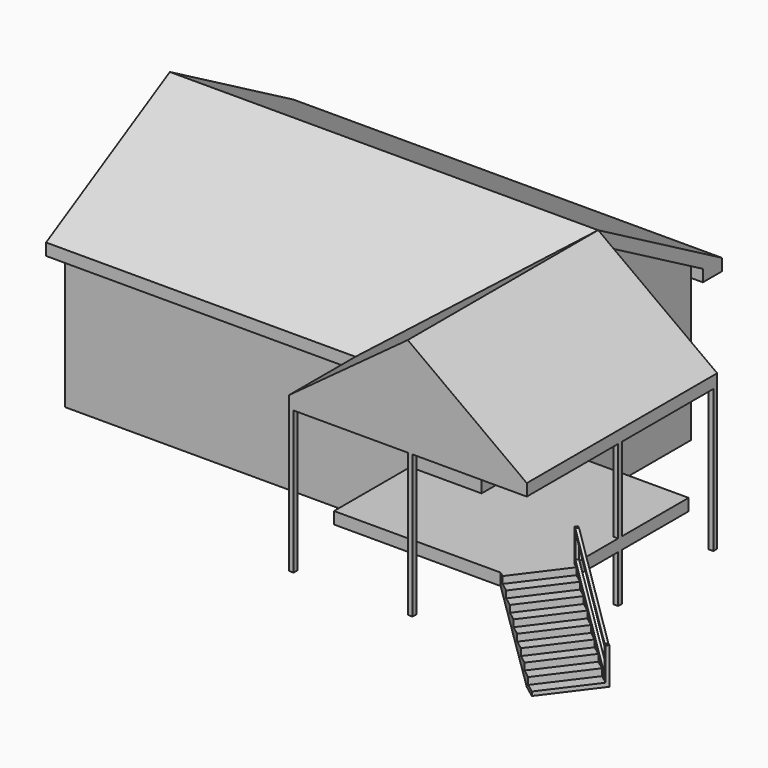
from build123d import *

# Parameters (mm, degrees)
F0_W           = 558.8
F0_H           = 304.8
F1_DEPTH       = 889
F3_DEPTH       = 889
F5_DEPTH       = 25.4
F7_DEPTH       = 330.2
F7_DEPTH_BACK  = 177.8
F8_W           = 10.16
F8_H           = 10.16
F9_DEPTH       = 304.8
F11_DEPTH      = 203.2
F11_DEPTH_BACK = 203.2
F14_DEPTH      = 25.4
F15_W          = 6.35
F15_H          = 127.005368185
F16_DEPTH      = 304.8
F18_DEPTH      = 25.4
F19_DEPTH      = 127
F20_W          = 6.5650812721
F20_H          = 95.2373991132
F21_DEPTH      = 6.35
F22_W          = 6.35
F22_H          = 78.3844
F23_DEPTH      = 6.35
F25_DEPTH      = 6.35
F27_DEPTH      = 6.35


# Not quite as in the source:
# - a feature of the source that left no trace in its solid (it failed there, or was rolled back) is left out


with BuildPart() as f1:
    # F0 (on Right) → F1 (new body)
    with BuildSketch(Plane.YZ):
        with Locations((279.4, -152.4)):
            Rectangle(F0_W, F0_H)
    extrude(amount=F1_DEPTH)

    # F2 (on face) → F3 (join)
    with BuildSketch(Plane(origin=(0, 0, 0), x_dir=(0, -1, 0), z_dir=(-1, 0, 0))):
        Polygon((-609.6, 0), (-558.8, 0), (0, 0), (50.8, 0), (50.8, 25.4), (-279.4, 211.5524560213), (-609.6, 25.4), align=None)
    extrude(amount=-F3_DEPTH)

    # F4 (on face) → F5 (join)
    with BuildSketch(Plane.YZ.offset(889)):
        Polygon((-50.8, 25.4), (-50.8, 0), (0, 0), (0, 25.4), (279.4, 182.9136166334), (558.8, 25.4), (558.8, 0), (609.6, 0), (609.6, 25.4), (279.4, 211.5524560213), align=None)
    extrude(amount=F5_DEPTH)

    # F6 (on face) → F7 (join, two sides)
    with BuildSketch(Plane.XZ.offset(50.8)) as f7_sk:
        Polygon((889, 0), (914.4, 0), (1168.4, 0), (1168.4, 25.4), (914.4, 211.6865664721), (660.4, 25.4), (660.4, 0), align=None)
    extrude(amount=-F7_DEPTH)
    extrude(f7_sk.sketch, amount=F7_DEPTH_BACK)

    # F8 (on face) → F9 (join)
    with BuildSketch(Plane(origin=(0, 0, 0), x_dir=(1, 0, 0), z_dir=(0, 0, -1))):
        with Locations((665.48, 223.52)):
            Rectangle(F8_W, F8_H)
        with Locations((1163.32, -274.32)):
            Rectangle(F8_W, F8_H)
        with Locations((1163.32, -20.32)):
            Rectangle(F8_W, F8_H)
        with Locations((919.48, 223.52)):
            Rectangle(F8_W, F8_H)
    extrude(amount=F9_DEPTH)

    # F10 (on face) → F11 (join, two sides)
    with BuildSketch(Plane.XZ) as f11_sk:
        Polygon((1168.4, -177.8), (889, -177.8), (736.6, -177.8), (736.6, -203.2), (1168.4, -203.2), align=None)
    extrude(amount=F11_DEPTH)
    extrude(f11_sk.sketch, amount=-F11_DEPTH_BACK)

    # F13 (on face) → F14 (cut)
    with BuildSketch(Plane.XY.offset(-177.8)):
        Polygon((1092.2, -203.2), (1168.4, -203.2), (1168.4, -101.6), align=None)
    extrude(amount=-F14_DEPTH, mode=Mode.SUBTRACT)

    # F15 (on face) → F16 (join)
    with BuildSketch(Plane(origin=(796.544, -597.408, 0), x_dir=(0.6, 0.8, 0), z_dir=(0.8, -0.6, 0))):
        with Locations((495.935, -241.3026840925)):
            Rectangle(F15_W, F15_H)
    extrude(amount=F16_DEPTH)

    # F17 (on face) → F18 (cut)
    with BuildSketch(Plane(origin=(295.656, 394.208, 0), x_dir=(0.8, -0.6, 0), z_dir=(-0.6, -0.8, 0))):
        Polygon((1170.1436042786, -304.805368185), (995.68, -203.2), (995.68, -304.805368185), align=None)
        Polygon((1300.48, -177.8), (1008.8101625443, -177.8), (1008.8101625443, -192.6082), (1033.2195625443, -192.6082), (1033.2195625443, -207.4164), (1057.6289625443, -207.4164), (1057.6289625443, -222.2246), (1082.0383625443, -222.2246), (1082.0383625443, -237.0328), (1106.4477625443, -237.0328), (1106.4477625443, -251.841), (1130.8571625443, -251.841), (1130.8571625443, -266.6492), (1155.2665625443, -266.6492), (1155.2665625443, -281.4574), (1179.6759625442, -281.4574), (1179.6759625442, -296.2656), (1204.0853625442, -296.2656), (1204.0853625442, -304.805368185), (1300.48, -304.805368185), align=None)
    extrude(amount=-F18_DEPTH, mode=Mode.SUBTRACT)

    # F19 (add): a face of the model
    f19_faces = [f1.faces().sort_by_distance(p)[0] for p in [
        (1167.2257565811, -259.4693174358, -245.1597520789),
    ]]
    extrude(f19_faces, amount=-F19_DEPTH)

    # F20 (on face) → F21 (join)
    with BuildSketch(Plane(origin=(371.856, 495.808, 0), x_dir=(-0.8, 0.6, 0), z_dir=(0.6, 0.8, 0))):
        with Locations((-998.9625406361, -155.5813004434)):
            Rectangle(F20_W, F20_H)
    extrude(amount=F21_DEPTH)

    # F22 (on face) → F23 (join)
    with BuildSketch(Plane(origin=(371.856, 495.808, 0), x_dir=(-0.8, 0.6, 0), z_dir=(0.6, 0.8, 0))):
        with Locations((-1200.9103625442, -265.613168185)):
            Rectangle(F22_W, F22_H)
    extrude(amount=F23_DEPTH)

    # F24 (on face) → F25 (join)
    with BuildSketch(Plane(origin=(375.666, 500.888, 0), x_dir=(-0.8, 0.6, 0), z_dir=(0.6, 0.8, 0))):
        Polygon((-1002.1302700043, -107.9991236329), (-1197.7353625442, -226.420968185), (-1197.7353625442, -232.770968185), (-1002.1302700043, -114.3491236329), align=None)
    extrude(amount=-F25_DEPTH)


with BuildPart() as f27:
    # F26 (on face) → F27 (new body)
    with BuildSketch(Plane(origin=(375.666, 500.888, 0), x_dir=(-0.8, 0.6, 0), z_dir=(0.6, 0.8, 0))):
        Polygon((-1002.2450812721, -166.8442318545), (-1197.7353625442, -285.196568185), (-1197.7353625442, -291.546568185), (-1002.2450812721, -173.1942318545), align=None)
    extrude(amount=-F27_DEPTH)


solid = Compound([f1.part, f27.part])
